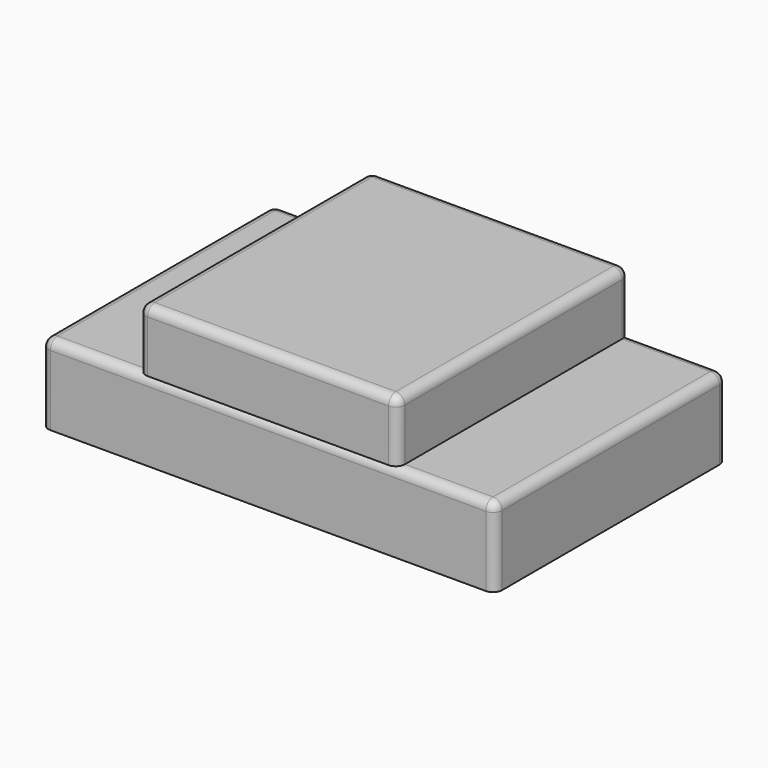
from build123d import *

# Parameters (mm, degrees)
F0_W            = 254.5158863068
F0_H            = 162.6137495041
F1_DEPTH        = 22.225
F2_W            = 145.3766971827
F2_H            = 162.6137495041
F3_DEPTH        = 34.29
F9_R            = 5.08
F10_R           = 5.08
F11_T1_DEPTH    = 170.2337495041
F11_T3_DEPTH    = 59.69
F11_S7_W        = 5.08
F11_S7_H        = 5.08
F11_T8_DEPTH    = 5.08
F12_T1_DEPTH    = 152.4537495041
F12_T3_DEPTH    = 52.07
F12_T5_DEPTH    = 262.1358863068
F12_S9_W        = 5.08
F12_S9_H        = 5.08
F12_T10_DEPTH   = 5.08
F12_S15_W       = 5.08
F12_S15_H       = 5.08
F12_T16_DEPTH   = 5.08
F13_T1_DEPTH    = 152.4537495041
F13_T3_DEPTH    = 41.91
F13_T5_DEPTH    = 135.2166971826
F13_S9_W        = 5.08
F13_S9_H        = 5.08
F13_T10_DEPTH   = 5.08
F13_S15_W       = 5.08
F13_S15_H       = 5.08
F13_T16_DEPTH   = 5.08
F13_S21_W       = 5.08
F13_S21_H       = 5.08
F13_T22_DEPTH   = 5.08
F13_2_T1_DEPTH  = 152.453749504
F13_2_T3_DEPTH  = 52.07
F13_2_S7_W      = 5.08
F13_2_S7_H      = 5.08
F13_2_T8_DEPTH  = 5.08
F13_2_T12_ANGLE = 90.0000000017
F14_W           = 21.5812288225
F14_H           = 10.1558715105
F15_DEPTH       = 5.08


# Not quite as in the source:
# - a fillet or chamfer that OpenCascade refuses, or shapes differently, is made with other operations: its cross-section is extruded or revolved along the edge and cut away or added


with BuildPart() as f1:
    # F0 (on Top) → F1 (new body, symmetric)
    with BuildSketch(Plane.XY):
        Rectangle(F0_W, F0_H)
    extrude(amount=F1_DEPTH, both=True)

    # F10
    f10_edges = [f1.edges().sort_by_distance(p)[0] for p in [
        (0, -81.306875, 22.225),
        (-127.257943, -81.306875, 0),
        (127.257943, -81.306875, 0),
    ]]
    fillet(f10_edges, radius=F10_R)

    # F12: fillet of radius 5.08 on 3 edges, made by hand

    # F12_s2 → F12_t1 (cut)
    with BuildSketch(Plane.XZ.offset(-76.226874752)):
        with BuildLine():
            ThreePointArc((-122.1779431534, 22.225), (-125.7700456018, 20.7371024484), (-127.2579431534, 17.145))
            Line((-127.2579431534, 17.145), (-127.2579431534, 22.225))
            Line((-127.2579431534, 22.225), (-122.1779431534, 22.225))
        make_face()
    extrude(amount=F12_T1_DEPTH, mode=Mode.SUBTRACT)

    # F12_s4 → F12_t3 (cut)
    with BuildSketch(Plane.XY.offset(-34.925)):
        with BuildLine():
            ThreePointArc((-122.1779431534, 81.306874752), (-125.7700456018, 79.8189772005), (-127.2579431534, 76.226874752))
            Line((-127.2579431534, 76.226874752), (-127.2579431534, 81.306874752))
            Line((-127.2579431534, 81.306874752), (-122.1779431534, 81.306874752))
        make_face()
    extrude(amount=F12_T3_DEPTH, mode=Mode.SUBTRACT)

    # F12_s6 → F12_t5 (cut)
    with BuildSketch(Plane.YZ.offset(-122.1779431534)):
        with BuildLine():
            ThreePointArc((81.306874752, 17.145), (79.8189772005, 20.7371024484), (76.226874752, 22.225))
            Line((76.226874752, 22.225), (81.306874752, 22.225))
            Line((81.306874752, 22.225), (81.306874752, 17.145))
        make_face()
    extrude(amount=F12_T5_DEPTH, mode=Mode.SUBTRACT)


with BuildPart() as f3:
    # F2 (on face) → F3 (new body)
    with BuildSketch(Plane.XY.offset(22.225)):
        Rectangle(F2_W, F2_H)
    extrude(amount=F3_DEPTH)

    # F9
    f9_edges = [f3.edges().sort_by_distance(p)[0] for p in [
        (0, -81.306875, 56.515),
        (-72.688349, -81.306875, 39.37),
        (72.688349, -81.306875, 39.37),
    ]]
    fillet(f9_edges, radius=F9_R)

    # F11: fillet of radius 5.08 on 2 edges, made by hand

    # F11_s2 → F11_t1 (cut)
    with BuildSketch(Plane.XZ.offset(-94.006874752)):
        with BuildLine():
            ThreePointArc((-72.6883485913, 51.435), (-71.2004510398, 55.0271024484), (-67.6083485913, 56.515))
            Line((-67.6083485913, 56.515), (-72.6883485913, 56.515))
            Line((-72.6883485913, 56.515), (-72.6883485913, 51.435))
        make_face()
    extrude(amount=F11_T1_DEPTH, mode=Mode.SUBTRACT)

    # F11_s4 → F11_t3 (cut)
    with BuildSketch(Plane.XY.offset(9.525)):
        with BuildLine():
            ThreePointArc((-72.6883485913, 76.226874752), (-71.2004510398, 79.8189772005), (-67.6083485913, 81.306874752))
            Line((-67.6083485913, 81.306874752), (-72.6883485913, 81.306874752))
            Line((-72.6883485913, 81.306874752), (-72.6883485913, 76.226874752))
        make_face()
    extrude(amount=F11_T3_DEPTH, mode=Mode.SUBTRACT)


with BuildPart() as f11_tool6:
    # F11_s7 → F11_t8 (new body)
    with BuildSketch(Plane.YZ.offset(-67.6083485913)):
        with Locations((-78.766874752, 53.975)):
            Rectangle(F11_S7_W, F11_S7_H)
    extrude(amount=-F11_T8_DEPTH)

    # F11_s9 → F11_t10 (revolve, cut)
    with BuildSketch(Plane(origin=(-67.6083485913, -76.226874752, 51.435), x_dir=(0, 0.7071067812, -0.7071067812), z_dir=(0, 0.7071067812, 0.7071067812))):
        with BuildLine():
            ThreePointArc((0, -5.08), (5.08, 0), (0, 5.08))
            Line((0, 5.08), (0, -5.08))
        make_face()
    revolve(axis=Axis((-67.6083485913, -76.226874752, 51.435), (-1, 0, 0)), mode=Mode.SUBTRACT)


with BuildPart() as f3_1:
    add(f3.part)

    # F11_t5: cut F11_tool6
    add(f11_tool6.part, mode=Mode.SUBTRACT)

    # F13: fillet of radius 5.08 on 3 edges, made by hand

    # F13_s2 → F13_t1 (cut)
    with BuildSketch(Plane.XZ.offset(-76.226874752)):
        with BuildLine():
            ThreePointArc((67.6083485913, 56.515), (71.2004510398, 55.0271024484), (72.6883485913, 51.435))
            Line((72.6883485913, 51.435), (72.6883485913, 56.515))
            Line((72.6883485913, 56.515), (67.6083485913, 56.515))
        make_face()
    extrude(amount=F13_T1_DEPTH, mode=Mode.SUBTRACT)

    # F13_s4 → F13_t3 (cut)
    with BuildSketch(Plane.XY.offset(9.525)):
        with BuildLine():
            ThreePointArc((67.6083485913, 81.306874752), (71.2004510398, 79.8189772005), (72.6883485913, 76.226874752))
            Line((72.6883485913, 76.226874752), (72.6883485913, 81.306874752))
            Line((72.6883485913, 81.306874752), (67.6083485913, 81.306874752))
        make_face()
    extrude(amount=F13_T3_DEPTH, mode=Mode.SUBTRACT)

    # F13_s6 → F13_t5 (cut)
    with BuildSketch(Plane.YZ.offset(-67.6083485913)):
        with BuildLine():
            ThreePointArc((76.226874752, 56.515), (79.8189772005, 55.0271024484), (81.306874752, 51.435))
            Line((81.306874752, 51.435), (81.306874752, 56.515))
            Line((81.306874752, 56.515), (76.226874752, 56.515))
        make_face()
    extrude(amount=F13_T5_DEPTH, mode=Mode.SUBTRACT)


with BuildPart() as f12_tool8:
    # F12_s9 → F12_t10 (new body)
    with BuildSketch(Plane.XY.offset(17.145)):
        with Locations((-124.7179431534, -78.766874752)):
            Rectangle(F12_S9_W, F12_S9_H)
    extrude(amount=F12_T10_DEPTH)

    # F12_s11 → F12_t12 (revolve, cut)
    with BuildSketch(Plane(origin=(-122.1779431534, -76.226874752, 17.145), x_dir=(0.7071067812, 0.7071067812, 0), z_dir=(0.7071067812, -0.7071067812, 0))):
        with BuildLine():
            ThreePointArc((0, -5.08), (5.08, 0), (0, 5.08))
            Line((0, 5.08), (0, -5.08))
        make_face()
    revolve(axis=Axis((-122.1779431534, -76.226874752, 17.145), (0, 0, 1)), mode=Mode.SUBTRACT)


with BuildPart() as f1_1:
    add(f1.part)

    # F12_t7: cut F12_tool8
    add(f12_tool8.part, mode=Mode.SUBTRACT)


with BuildPart() as f12_tool14:
    # F12_s15 → F12_t16 (new body)
    with BuildSketch(Plane.XZ.offset(-76.226874752)):
        with Locations((-124.7179431534, 19.685)):
            Rectangle(F12_S15_W, F12_S15_H)
    extrude(amount=-F12_T16_DEPTH)

    # F12_s17 → F12_t18 (revolve, cut)
    with BuildSketch(Plane(origin=(-122.1779431534, 76.226874752, 17.145), x_dir=(0.7071067812, 0, -0.7071067812), z_dir=(0.7071067812, 0, 0.7071067812))):
        with BuildLine():
            ThreePointArc((0, -5.08), (5.08, 0), (0, 5.08))
            Line((0, 5.08), (0, -5.08))
        make_face()
    revolve(axis=Axis((-122.1779431534, 76.226874752, 17.145), (0, 1, 0)), mode=Mode.SUBTRACT)


with BuildPart() as f1_2:
    add(f1_1.part)

    # F12_t13: cut F12_tool14
    add(f12_tool14.part, mode=Mode.SUBTRACT)

    # F13#2: fillet of radius 5.08 on 1 edges, made by hand

    # F13_2_s2 → F13_2_t1 (cut)
    with BuildSketch(Plane.XZ.offset(-76.226874752)):
        with BuildLine():
            ThreePointArc((127.2579431534, 17.145), (125.7700456018, 20.7371024484), (122.1779431534, 22.225))
            Line((122.1779431534, 22.225), (127.2579431534, 22.225))
            Line((127.2579431534, 22.225), (127.2579431534, 17.145))
        make_face()
    extrude(amount=F13_2_T1_DEPTH, mode=Mode.SUBTRACT)

    # F13_2_s4 → F13_2_t3 (cut)
    with BuildSketch(Plane.XY.offset(-34.925)):
        with BuildLine():
            ThreePointArc((127.2579431534, 76.226874752), (125.7700456018, 79.8189772005), (122.1779431534, 81.306874752))
            Line((122.1779431534, 81.306874752), (127.2579431534, 81.306874752))
            Line((127.2579431534, 81.306874752), (127.2579431534, 76.226874752))
        make_face()
    extrude(amount=F13_2_T3_DEPTH, mode=Mode.SUBTRACT)


with BuildPart() as f13_tool8:
    # F13_s9 → F13_t10 (new body)
    with BuildSketch(Plane.XY.offset(51.435)):
        with Locations((-70.1483485913, 78.766874752)):
            Rectangle(F13_S9_W, F13_S9_H)
    extrude(amount=F13_T10_DEPTH)

    # F13_s11 → F13_t12 (revolve, cut)
    with BuildSketch(Plane(origin=(-67.6083485913, 76.226874752, 51.435), x_dir=(0.7071067812, -0.7071067812, 0), z_dir=(-0.7071067812, -0.7071067812, 0))):
        with BuildLine():
            ThreePointArc((0, -5.08), (5.08, 0), (0, 5.08))
            Line((0, 5.08), (0, -5.08))
        make_face()
    revolve(axis=Axis((-67.6083485913, 76.226874752, 51.435), (0, 0, 1)), mode=Mode.SUBTRACT)


with BuildPart() as f3_2:
    add(f3_1.part)

    # F13_t7: cut F13_tool8
    add(f13_tool8.part, mode=Mode.SUBTRACT)


with BuildPart() as f13_tool14:
    # F13_s15 → F13_t16 (new body)
    with BuildSketch(Plane.XY.offset(51.435)):
        with Locations((70.1483485913, -78.766874752)):
            Rectangle(F13_S15_W, F13_S15_H)
    extrude(amount=F13_T16_DEPTH)

    # F13_s17 → F13_t18 (revolve, cut)
    with BuildSketch(Plane(origin=(67.6083485913, -76.226874752, 51.435), x_dir=(-0.7071067812, 0.7071067812, 0), z_dir=(0.7071067812, 0.7071067812, 0))):
        with BuildLine():
            ThreePointArc((0, -5.08), (5.08, 0), (0, 5.08))
            Line((0, 5.08), (0, -5.08))
        make_face()
    revolve(axis=Axis((67.6083485913, -76.226874752, 51.435), (0, 0, 1)), mode=Mode.SUBTRACT)


with BuildPart() as f3_3:
    add(f3_2.part)

    # F13_t13: cut F13_tool14
    add(f13_tool14.part, mode=Mode.SUBTRACT)


with BuildPart() as f13_tool20:
    # F13_s21 → F13_t22 (new body)
    with BuildSketch(Plane.XZ.offset(-76.226874752)):
        with Locations((70.1483485913, 53.975)):
            Rectangle(F13_S21_W, F13_S21_H)
    extrude(amount=-F13_T22_DEPTH)

    # F13_s23 → F13_t24 (revolve, cut)
    with BuildSketch(Plane(origin=(67.6083485913, 76.226874752, 51.435), x_dir=(-0.7071067812, 0, -0.7071067812), z_dir=(0.7071067812, 0, -0.7071067812))):
        with BuildLine():
            ThreePointArc((0, -5.08), (5.08, 0), (0, 5.08))
            Line((0, 5.08), (0, -5.08))
        make_face()
    revolve(axis=Axis((67.6083485913, 76.226874752, 51.435), (0, 1, 0)), mode=Mode.SUBTRACT)


with BuildPart() as f3_4:
    add(f3_3.part)

    # F13_t19: cut F13_tool20
    add(f13_tool20.part, mode=Mode.SUBTRACT)


with BuildPart() as f13_2_tool6:
    # F13_2_s7 → F13_2_t8 (new body)
    with BuildSketch(Plane.YZ.offset(122.1779431534)):
        with Locations((-78.766874752, 19.685)):
            Rectangle(F13_2_S7_W, F13_2_S7_H)
    extrude(amount=F13_2_T8_DEPTH)

    # F13_2_s9 → F13_2_t10 (revolve, cut)
    with BuildSketch(Plane(origin=(122.1779431534, -76.226874752, 17.145), x_dir=(0, 0.7071067812, -0.7071067812), z_dir=(0, -0.7071067812, -0.7071067812))):
        with BuildLine():
            ThreePointArc((0, -5.08), (5.08, 0), (0, 5.08))
            Line((0, 5.08), (0, -5.08))
        make_face()
    revolve(axis=Axis((122.1779431534, -76.226874752, 17.145), (1, 0, 0)), mode=Mode.SUBTRACT)


with BuildPart() as f1_3:
    add(f1_2.part)

    # F13_2_t5: cut F13_2_tool6
    add(f13_2_tool6.part, mode=Mode.SUBTRACT)

    # F13_2_s11 → F13_2_t12 (revolve, cut)
    with BuildSketch(Plane.XZ.offset(-76.2268747521)):
        with BuildLine():
            ThreePointArc((127.2579431534, 17.145), (125.7700456018, 20.7371024484), (122.1779431534, 22.225))
            Line((122.1779431534, 22.225), (127.2579431534, 22.225))
            Line((127.2579431534, 22.225), (127.2579431534, 17.145))
        make_face()
    revolve(axis=Axis((127.2579431534, 76.2268747521, 17.1450000001), (-1, 0, 0)), revolution_arc=F13_2_T12_ANGLE, mode=Mode.SUBTRACT)

    # F14 (on face) → F15 (join)
    with BuildSketch(Plane(origin=(-127.2579431534, 0, 0), x_dir=(0, -1, 0), z_dir=(-1, 0, 0))):
        with Locations((-59.269035235, 8.1159230322)):
            Rectangle(F14_W, F14_H)
        with Locations((58.9516628534, 8.1159230322)):
            Rectangle(F14_W, F14_H)
    extrude(amount=F15_DEPTH)


solid = Compound([f3_4.part, f1_3.part])
